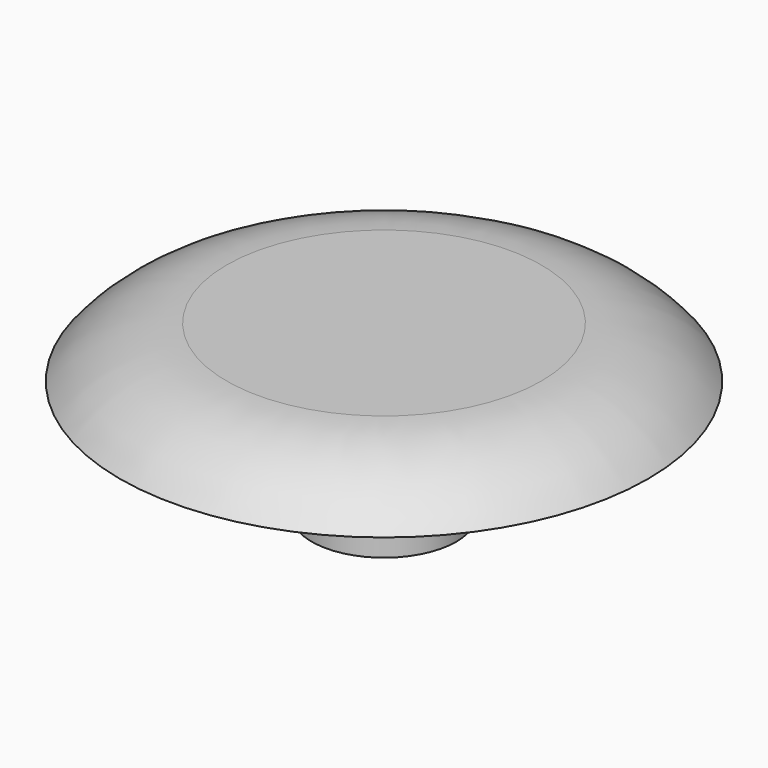
from build123d import *

# Parameters (mm, degrees)
F0_R     = 9.806931969
F0_R_2   = 2.6876925043
F1_DEPTH = 1.905
F2_DEPTH = 4.3688


# Not quite as in the source:
# - a fillet or chamfer that OpenCascade refuses, or shapes differently, is made with other operations: its cross-section is extruded or revolved along the edge and cut away or added


with BuildPart() as f1:
    # F0 (on Top) → F1 (new body)
    with BuildSketch(Plane.XY):
        Circle(F0_R)
        Circle(F0_R_2, mode=Mode.SUBTRACT)
        Circle(F0_R_2)
    extrude(amount=F1_DEPTH)

    # F0 (on Top) → F2 (join)
    with BuildSketch(Plane.XY):
        Circle(F0_R_2)
    extrude(amount=-F2_DEPTH)

    # F3: fillet of radius 5.08 on 1 edges, made by hand

    # F3_s1 → F3_t2 (revolve, cut)
    with BuildSketch(Plane.XZ):
        with BuildLine():
            ThreePointArc((9.806931969, 0), (8.0410627657, 1.4040501198), (5.8413582401, 1.905))
            Line((5.8413582401, 1.905), (9.806931969, 1.905))
            Line((9.806931969, 1.905), (9.806931969, 0))
        make_face()
    revolve(axis=Axis((0, 0, 1.905), (0, 0, 1)), mode=Mode.SUBTRACT)


solid = f1.part
